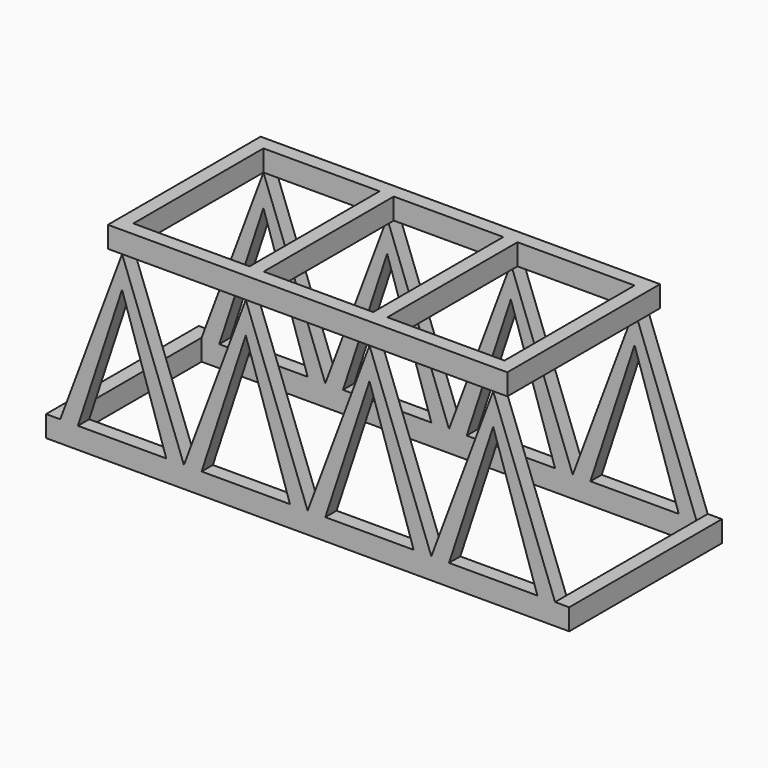
from build123d import *

# Parameters (mm, degrees)
F0_W      = 177.8
F0_H      = 7.62
F1_DEPTH  = 5.08
F0_W_2    = 133.35
F3_DEPTH  = 5.08
F4_W      = 58.42
F4_H      = 7.62
F4_W_2    = 5.08
F5_DEPTH  = 5.08
F6_W      = 182.88
F6_H      = 7.62
F7_DEPTH  = 5.08
F8_W      = 68.6033219099
F8_H      = 7.62
F9_DEPTH  = 5.08
F11_DEPTH = 5.08
F12_W     = 63.5
F12_H     = 7.62
F13_DEPTH = 5.08
F14_W     = 138.43
F14_H     = 7.62
F15_DEPTH = 5.08
F16_W     = 68.58
F16_H     = 7.62
F17_DEPTH = 5.08
F18_W     = 5.08
F18_H     = 7.62
F19_DEPTH = 63.5
F20_W     = 5.08
F20_H     = 7.62
F21_DEPTH = 63.5


# Not quite as in the source:
# - a pattern or mirror of a feature is missing from the dataset's text; its kind, count and spacing are read off the source's solid


with BuildPart() as f1:
    # F0 (on Front) → F1 (new body)
    with BuildSketch(Plane.XZ):
        with Locations((0, -38.8273451847)):
            Rectangle(F0_W, F0_H)
    extrude(amount=-F1_DEPTH)

    # F2 (on Front) → F3 (join)
    with BuildSketch(Plane.XZ):
        Polygon((-66.675, 24.46626075), (-88.9, -35.0173451847), (-82.55, -35.0173451847), (-66.675, 13.2384770029), (-50.8, -35.0173451847), (-44.45, -35.0173451847), align=None)
        Polygon((-22.225, 24.46626075), (-44.45, -35.0173451847), (-38.1, -35.0173451847), (-22.225, 13.2384770029), (-6.35, -35.0173451847), (0, -35.0173451847), align=None)
        Polygon((22.225, 24.46626075), (0, -35.0173451847), (6.35, -35.0173451847), (22.225, 13.2384770029), (38.1, -35.0173451847), (44.45, -35.0173451847), align=None)
        Polygon((66.675, 24.46626075), (44.45, -35.0173451847), (50.8, -35.0173451847), (66.675, 13.2384770029), (82.55, -35.0173451847), (88.9, -35.0173451847), align=None)
    f3 = extrude(amount=-F3_DEPTH)

    # F3_copies: F3 across plane
    add(f3.mirror(Plane.ZX.offset(34.29)))

    # F4 (on face) → F5 (join)
    with BuildSketch(Plane(origin=(-88.9, 0, 0), x_dir=(0, -1, 0), z_dir=(-1, 0, 0))):
        with Locations((-34.29, -38.8273451847)):
            Rectangle(F4_W, F4_H)
        with Locations((-2.54, -38.8273451847)):
            Rectangle(F4_W_2, F4_H)
    extrude(amount=F5_DEPTH)

    # F6 (on face) → F7 (join)
    with BuildSketch(Plane(origin=(0, 63.5, 0), x_dir=(-1, 0, 0), z_dir=(0, 1, 0))):
        with Locations((2.54, -38.8273451847)):
            Rectangle(F6_W, F6_H)
    extrude(amount=F7_DEPTH)

    # F8 (on face) → F9 (join)
    with BuildSketch(Plane.YZ.offset(88.9)):
        with Locations((34.301660955, -38.8273451847)):
            Rectangle(F8_W, F8_H)
    extrude(amount=F9_DEPTH)

    # F10 (on face) → F11 (join)
    with BuildSketch(Plane.XZ):
        Polygon((-66.675, 24.46626075), (-88.9, -35.0173451847), (-82.55, -35.0173451847), (-66.675, 13.2384770029), (-50.8, -35.0173451847), (-44.45, -35.0173451847), align=None)
        Polygon((-22.225, 24.46626075), (-44.45, -35.0173451847), (-38.1, -35.0173451847), (-22.225, 13.2384770029), (-6.35, -35.0173451847), (0, -35.0173451847), align=None)
        Polygon((22.225, 24.46626075), (0, -35.0173451847), (6.35, -35.0173451847), (22.225, 13.2384770029), (38.1, -35.0173451847), (44.45, -35.0173451847), align=None)
        Polygon((82.55, -35.0173451847), (88.9, -35.0173451847), (66.675, 24.46626075), (44.45, -35.0173451847), (50.8, -35.0173451847), (66.675, 13.2384770029), align=None)
    extrude(amount=-F11_DEPTH)


with BuildPart() as f1b:
    # F0 (on Front) → F1, piece 2 (new body)
    with BuildSketch(Plane.XZ):
        with Locations((0, 28.2794548153)):
            Rectangle(F0_W_2, F0_H)
    extrude(amount=-F1_DEPTH)

    # F12 (on face) → F13 (join)
    with BuildSketch(Plane.YZ.offset(66.675)):
        with Locations((31.75, 28.2794548153)):
            Rectangle(F12_W, F12_H)
    extrude(amount=F13_DEPTH)

    # F14 (on face) → F15 (join)
    with BuildSketch(Plane(origin=(0, 63.5, 0), x_dir=(-1, 0, 0), z_dir=(0, 1, 0))):
        with Locations((-2.54, 28.2794548153)):
            Rectangle(F14_W, F14_H)
    extrude(amount=F15_DEPTH)

    # F16 (on face) → F17 (join)
    with BuildSketch(Plane(origin=(-66.675, 0, 0), x_dir=(0, -1, 0), z_dir=(-1, 0, 0))):
        with Locations((-34.29, 28.2794548153)):
            Rectangle(F16_W, F16_H)
    extrude(amount=F17_DEPTH)

    # F18 (on face) → F19 (join)
    with BuildSketch(Plane.XZ.offset(-63.5)):
        with Locations((-22.3953099983, 28.2794548153)):
            Rectangle(F18_W, F18_H)
    extrude(amount=F19_DEPTH)

    # F20 (on face) → F21 (join)
    with BuildSketch(Plane.XZ.offset(-63.5)):
        with Locations((22.0546900017, 28.2794548153)):
            Rectangle(F20_W, F20_H)
    extrude(amount=F21_DEPTH)


solid = Compound([f1.part, f1b.part])
